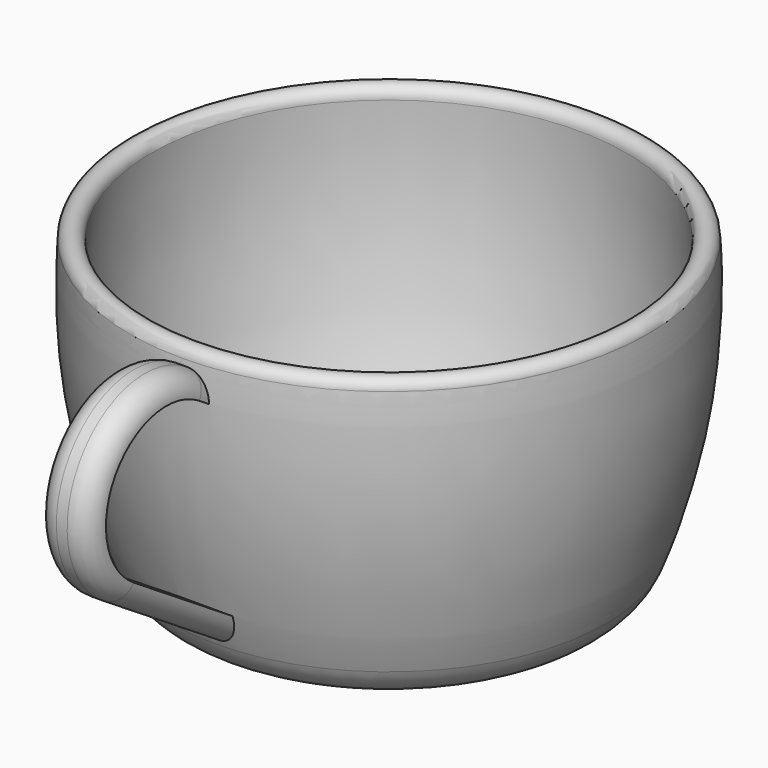
from build123d import *

# Parameters (mm, degrees)
F4_W = 5
F4_H = 2
F7_R = 1.99999


# Not quite as in the source:
# - a fillet or chamfer is up to 0.001 mm smaller than in the source, because OpenCascade refuses the exact size


with BuildPart() as f1:
    # F0 (on Right) → F1 (revolve)
    with BuildSketch(Plane.YZ):
        with BuildLine():
            Line((-15.5, 0), (0, 0))
            Line((0, 0), (0, 2))
            Line((0, 2), (-14.1140147466, 2))
            ThreePointArc((-14.1140147466, 2), (-16.9895559094, 2.9096133409), (-18.8188448306, 5.3074947916))
            ThreePointArc((-18.8188448306, 5.3074947916), (-21.5779187909, 16.4567716512), (-22.0043016514, 27.9344483005))
            ThreePointArc((-22.0043016514, 27.9344483005), (-22.9365991261, 28.9978491743), (-24, 28.0655516995))
            ThreePointArc((-24, 28.0655516995), (-23.4455119823, 15.4131291908), (-20.1580426519, 3.1826836674))
            ThreePointArc((-20.1580426519, 3.1826836674), (-18.3207639335, 0.8716479279), (-15.5, 0))
        make_face()
    revolve(axis=Axis((0, 0, 12.4431038275), (0, 0, 1)))

    # F4 (on line) → F5 (join, up to the next surface of F1)
    with BuildSketch(Plane(origin=(0, -29.4754881711, 19.1533482092), x_dir=(-1, 0, 0), z_dir=(0, 0.8385179515, -0.5448739716))):
        with Locations((0, 8.9890159432)):
            Rectangle(F4_W, F4_H)
    extrude(until=Until.NEXT)

    # F6: sweep along a path in F2
    with BuildLine(Plane.YZ) as f6_path:
        ThreePointArc((-24.0327333815, 27.5293173957), (-36.4908432768, 24.8748327821), (-33.8170755575, 12.4208471988))
        Line((-33.8170755575, 12.4208471988), (-20.3738602098, 3.7444446542))
    # F4 (on line) → F6 (sweep)
    with BuildSketch(Plane(origin=(0, -29.4754881711, 19.1533482092), x_dir=(-1, 0, 0), z_dir=(0, 0.8385179515, -0.5448739716))):
        with Locations((0, 8.9890159432)):
            Rectangle(F4_W, F4_H)
    sweep(path=f6_path.line)

    # F7 (radius 2 in the source; OpenCascade refuses exactly that, so slightly less here)
    f7_edges = [f1.edges().sort_by_distance(p)[0] for p in [
        (-2.5, -36.490843, 24.874833),
        (2.5, -36.490843, 24.874833),
    ]]
    fillet(f7_edges, radius=F7_R)


solid = f1.part
